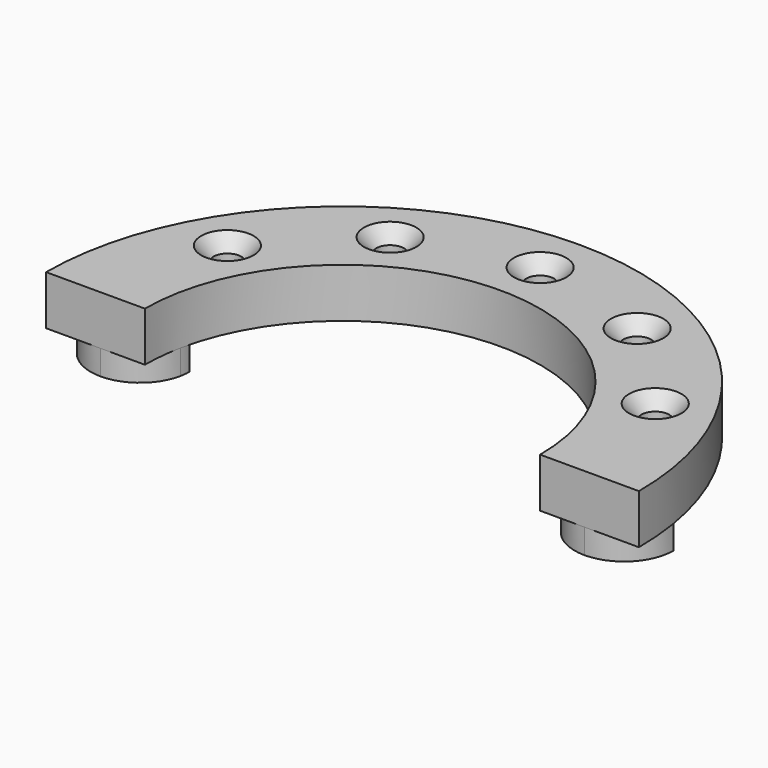
from build123d import *

# Parameters (mm, degrees)
F1_DEPTH       = 12.7
F3_DEPTH       = 6.35
F5_D           = 7.1374
F5_CSINK_D     = 13.4874
F5_CSINK_ANGLE = 82


with BuildPart() as f1:
    # F0 (on Top) → F1 (new body)
    with BuildSketch(Plane.XY):
        with BuildLine():
            Line((-76.2, 0), (-50.8, 0))
            ThreePointArc((-50.8, 0), (0, 50.8), (50.8, 0))
            Line((50.8, 0), (76.2, 0))
            ThreePointArc((76.2, 0), (0, 76.2), (-76.2, 0))
        make_face()
    extrude(amount=F1_DEPTH)

    # F2 (on face) → F3 (join)
    with BuildSketch(Plane(origin=(0, 0, 0), x_dir=(1, 0, 0), z_dir=(0, 0, -1))):
        with BuildLine():
            Line((-74.9170394667, -12.7), (-49.5170394667, -12.7))
            ThreePointArc((-49.5170394667, -12.7), (-49.581350313, -11.4235362865), (-49.7736315316, -10.1600002047))
            ThreePointArc((-49.7736315316, -10.1600002047), (-54.1848541289, -2.8626223667), (-62.2170394667, 0))
            ThreePointArc((-62.2170394667, 0), (-71.1972955878, -3.7197438789), (-74.9170394667, -12.7))
        make_face()
        with BuildLine():
            ThreePointArc((62.2170394667, 0), (54.1848541308, -2.8626223652), (49.7736315325, -10.1600001999))
            ThreePointArc((49.7736315325, -10.1600001999), (49.5813503133, -11.423536284), (49.5170394667, -12.7))
            Line((49.5170394667, -12.7), (74.9170394667, -12.7))
            ThreePointArc((74.9170394667, -12.7), (71.1972955878, -3.7197438789), (62.2170394667, 0))
        make_face()
    extrude(amount=F3_DEPTH)

    # F5 (through all)
    with Locations(Plane.XY.offset(12.7)):
        with Locations((-54.9926131403, 31.75), (-31.75, 54.9926131403), (0, 63.5), (31.75, 54.9926131403), (54.9926131403, 31.75)):
            CounterSinkHole(F5_D / 2, F5_CSINK_D / 2, counter_sink_angle=F5_CSINK_ANGLE)


solid = f1.part
